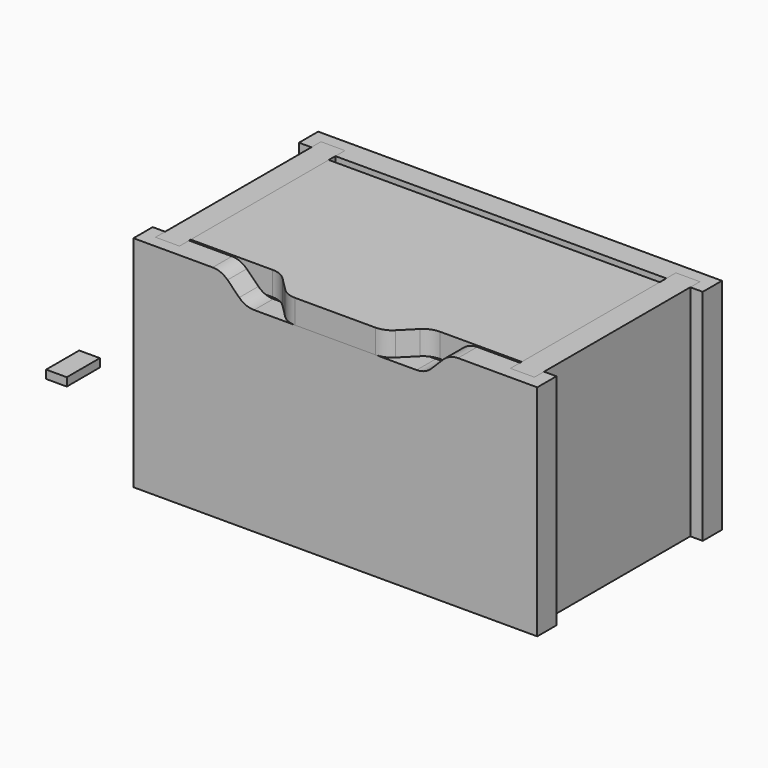
from build123d import *

# Parameters (mm, degrees)
F6_DEPTH      = 50
F6_DEPTH_BACK = 3
F5_W          = 5.8
F5_H          = 2.9
F5_H_2        = 44.2
F7_DEPTH      = 50
F7_DEPTH_BACK = 3
F5_W_2        = 80
F8_DEPTH      = 5.8
F9_W          = 85.8
F9_H          = 50
F9_W_2        = 83.8
F9_H_2        = 48
F9_W_3        = 80
F9_H_3        = 44.2
F10_DEPTH     = 3.675
F11_DEPTH     = 3.375
F13_DEPTH     = 5.8
F15_DEPTH     = 25.4
F16_R         = 5.08
F16_2_R       = 5.08
F17_W         = 5
F17_H         = 10
F18_DEPTH     = 2


# Not quite as in the source:
# - a length typed as a fraction of an inch, garbled in the dataset ("3 / 203.2 mm" for 3/8 in), is restored


with BuildPart() as f6:
    # F5 (on Top) → F6 (new body, two sides)
    with BuildSketch(Plane.XY) as f6_sk:
        Polygon((-48.8, 22.1), (-45.8, 22.1), (-45.8, 25), (-40, 25), (-40, 22.1), (40, 22.1), (40, 25), (45.8, 25), (45.8, 22.1), (48.8, 22.1), (48.8, 27.9), (-48.8, 27.9), align=None)
    extrude(amount=F6_DEPTH)
    extrude(f6_sk.sketch, amount=-F6_DEPTH_BACK)


with BuildPart() as f6b:
    # F5 (on Top) → F6, piece 2 (new body, two sides)
    with BuildSketch(Plane.XY) as f6_2_sk:
        Polygon((-45.8, -25), (-45.8, -22.1), (-48.8, -22.1), (-48.8, -27.9), (48.8, -27.9), (48.8, -22.1), (45.8, -22.1), (45.8, -25), (40, -25), (40, -22.1), (-40, -22.1), (-40, -25), align=None)
    extrude(amount=F6_DEPTH)
    extrude(f6_2_sk.sketch, amount=-F6_DEPTH_BACK)


with BuildPart() as f7:
    # F5 (on Top) → F7 (new body, two sides)
    with BuildSketch(Plane.XY) as f7_sk:
        with Locations((-42.9, 23.55)):
            Rectangle(F5_W, F5_H)
        with Locations((-42.9, 0)):
            Rectangle(F5_W, F5_H_2)
        with Locations((-42.9, -23.55)):
            Rectangle(F5_W, F5_H)
    extrude(amount=F7_DEPTH)
    extrude(f7_sk.sketch, amount=-F7_DEPTH_BACK)


with BuildPart() as f7b:
    # F5 (on Top) → F7, piece 2 (new body, two sides)
    with BuildSketch(Plane.XY) as f7_2_sk:
        with Locations((42.9, 23.55)):
            Rectangle(F5_W, F5_H)
        with Locations((42.9, 0)):
            Rectangle(F5_W, F5_H_2)
        with Locations((42.9, -23.55)):
            Rectangle(F5_W, F5_H)
    extrude(amount=F7_DEPTH)
    extrude(f7_2_sk.sketch, amount=-F7_DEPTH_BACK)


with BuildPart() as f8:
    # F5 (on Top) → F8 (new body)
    with BuildSketch(Plane.XY):
        Rectangle(F5_W_2, F5_H_2)
    extrude(amount=F8_DEPTH)

    # F9 (on face) → F11 (join)
    with BuildSketch(Plane.XY.offset(5.8)):
        Rectangle(F9_W_2, F9_H_2)
        Rectangle(F9_W_3, F9_H_3, mode=Mode.SUBTRACT)
    extrude(amount=-F11_DEPTH)


with BuildPart() as f10_tool:
    # F9 (on face) → F10 (new body)
    with BuildSketch(Plane.XY.offset(5.8)):
        Rectangle(F9_W, F9_H)
        Rectangle(F9_W_2, F9_H_2, mode=Mode.SUBTRACT)
        Rectangle(F9_W_2, F9_H_2)
        Rectangle(F9_W_3, F9_H_3, mode=Mode.SUBTRACT)
    extrude(amount=-F10_DEPTH)


with BuildPart() as f6_1:
    add(f6.part)

    # F10: cut by f10_tool
    add(f10_tool.part, mode=Mode.SUBTRACT)


with BuildPart() as f6b_1:
    add(f6b.part)

    # F10: cut by f10_tool
    add(f10_tool.part, mode=Mode.SUBTRACT)

    # F14 (on face) → F15 (cut)
    with BuildSketch(Plane.XZ.offset(27.9)):
        Polygon((0, 50), (-27.5484826416, 50), (-21.7484826416, 44.2), (0, 44.2), (21.7484826416, 44.2), (27.5484826416, 50), align=None)
    extrude(amount=-F15_DEPTH, mode=Mode.SUBTRACT)

    # F16
    f16_edges = [f6b_1.edges().sort_by_distance(p)[0] for p in [
        (-27.548483, -25, 50),
        (-21.748483, -25, 44.2),
        (21.748483, -25, 44.2),
        (27.548483, -25, 50),
    ]]
    fillet(f16_edges, radius=F16_R)


with BuildPart() as f7_1:
    add(f7.part)

    # F10: cut by f10_tool
    add(f10_tool.part, mode=Mode.SUBTRACT)


with BuildPart() as f7b_1:
    add(f7b.part)

    # F10: cut by f10_tool
    add(f10_tool.part, mode=Mode.SUBTRACT)


with BuildPart() as f13:
    # F12 (on face) → F13 (new body)
    with BuildSketch(Plane.XY.offset(50)):
        Polygon((40, 20.1), (-40, 20.1), (-40, -21.6), (-18.1196574122, -21.6), (-11.8196574122, -27.9), (0, -27.9), (11.8196574122, -27.9), (18.1196574122, -21.6), (40, -21.6), align=None)
    extrude(amount=-F13_DEPTH)

    # F16#2
    f16_2_edges = [f13.edges().sort_by_distance(p)[0] for p in [
        (18.119657, -21.6, 47.1),
        (11.819657, -27.9, 47.1),
        (-11.819657, -27.9, 47.1),
        (-18.119657, -21.6, 47.1),
    ]]
    fillet(f16_2_edges, radius=F16_2_R)


with BuildPart() as f18:
    # F17 (on Top) → F18 (new body)
    with BuildSketch(Plane.XY):
        with Locations((-83.2338705659, -3.1428090297)):
            Rectangle(F17_W, F17_H)
    extrude(amount=F18_DEPTH)


solid = Compound([f8.part, f6_1.part, f6b_1.part, f7_1.part, f7b_1.part, f13.part, f18.part])
